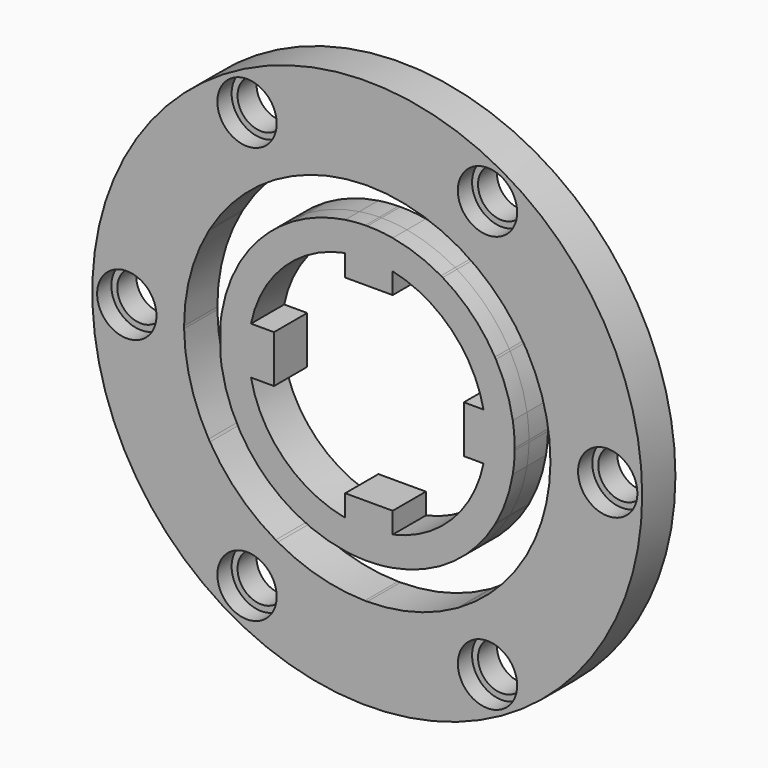
from build123d import *

# Parameters (mm, degrees)
F1_DEPTH      = 1.5
F1_DEPTH_BACK = 2
F0_R          = 23.1715188415
F14_D         = 4
F14_DEPTH     = 2.001
F15_D         = 5
F15_DEPTH     = 2
F15_TIP       = 1.5021515476


# Not quite as in the source:
# - the program builds the solid bodies; features that only make, move or delete a surface that nothing else refers to are left out


with BuildPart() as f1:
    # F0 (on Front) → F1 (new body, two sides)
    with BuildSketch(Plane.XZ) as f1_sk:
        with BuildLine():
            ThreePointArc((-9.7979589711, 2), (-7.0199538443, 7.1218149389), (-1.8586532747, 9.8257522869))
            Line((-1.8586532747, 9.8257522869), (-1.8586532747, 12.2861632234))
            ThreePointArc((-1.8586532747, 12.2861632234), (-4.1072121765, 11.7275405301), (-6.2129783266, 10.761194128))
            ThreePointArc((-6.2129783266, 10.761194128), (-6.2850915316, 10.7161183391), (-6.3596317791, 10.6751806721))
            ThreePointArc((-6.3596317791, 10.6751806721), (-8.7864782122, 8.7864782122), (-10.6751806721, 6.3596317791))
            ThreePointArc((-10.6751806721, 6.3596317791), (-10.7161183391, 6.2850915316), (-10.761194128, 6.2129783266))
            ThreePointArc((-10.761194128, 6.2129783266), (-11.7036993668, 4.174664044), (-12.2639471113, 2))
            Line((-12.2639471113, 2), (-9.7979589711, 2))
        make_face()
        with BuildLine():
            ThreePointArc((-9.7979589711, -2), (-10, 0), (-9.7979589711, 2))
            Line((-9.7979589711, 2), (-12.2639471113, 2))
            ThreePointArc((-12.2639471113, 2), (-12.3163951558, 1.6464534963), (-12.3586532747, 1.2915448051))
            Line((-12.3586532747, 1.2915448051), (-12.3586532747, -1.2915448051))
            ThreePointArc((-12.3586532747, -1.2915448051), (-12.3163951558, -1.6464534963), (-12.2639471113, -2))
            Line((-12.2639471113, -2), (-9.7979589711, -2))
        make_face()
        with BuildLine():
            Line((-7.8586532747, 2), (-9.7979589711, 2))
            ThreePointArc((-9.7979589711, 2), (-10, 0), (-9.7979589711, -2))
            Line((-9.7979589711, -2), (-7.8586532747, -2))
            Line((-7.8586532747, -2), (-7.8586532747, 2))
        make_face()
        with BuildLine():
            Line((-1.8586532747, -12.2861632234), (-1.8586532747, -9.8257522869))
            ThreePointArc((-1.8586532747, -9.8257522869), (-7.0199538443, -7.1218149389), (-9.7979589711, -2))
            Line((-9.7979589711, -2), (-12.2639471113, -2))
            ThreePointArc((-12.2639471113, -2), (-11.7036993668, -4.174664044), (-10.761194128, -6.2129783266))
            ThreePointArc((-10.761194128, -6.2129783266), (-10.7161183391, -6.2850915316), (-10.6751806721, -6.3596317791))
            ThreePointArc((-10.6751806721, -6.3596317791), (-8.7261627517, -8.8463824459), (-6.2129783266, -10.761194128))
            ThreePointArc((-6.2129783266, -10.761194128), (-6.1378849458, -10.801108101), (-6.0651617625, -10.8451930155))
            ThreePointArc((-6.0651617625, -10.8451930155), (-4.02688589, -11.7553642554), (-1.8586532747, -12.2861632234))
        make_face()
        with BuildLine():
            Line((2.1413467253, -12.2400585354), (2.1413467253, -9.7680414722))
            ThreePointArc((2.1413467253, -9.7680414722), (0.144262023, -9.9989593693), (-1.8586532747, -9.8257522869))
            Line((-1.8586532747, -9.8257522869), (-1.8586532747, -12.2861632234))
            ThreePointArc((-1.8586532747, -12.2861632234), (-1.0166984011, -12.3842934037), (-0.1700123434, -12.4247935416))
            ThreePointArc((-0.1700123434, -12.4247935416), (-0.0849897619, -12.4229764774), (0, -12.4259566532))
            ThreePointArc((0, -12.4259566532), (1.0747004127, -12.3793948871), (2.1413467253, -12.2400585354))
        make_face()
        with BuildLine():
            ThreePointArc((-1.8586532747, -9.8257522869), (0.144262023, -9.9989593693), (2.1413467253, -9.7680414722))
            Line((2.1413467253, -9.7680414722), (2.1413467253, -8))
            Line((2.1413467253, -8), (-1.8586532747, -8))
            Line((-1.8586532747, -8), (-1.8586532747, -9.8257522869))
        make_face()
        with BuildLine():
            Line((12.2639471113, -2), (9.7979589711, -2))
            ThreePointArc((9.7979589711, -2), (7.1219640694, -7.0198025466), (2.1413467253, -9.7680414722))
            Line((2.1413467253, -9.7680414722), (2.1413467253, -12.2400585354))
            ThreePointArc((2.1413467253, -12.2400585354), (4.1621037763, -11.708171971), (6.0651617625, -10.8451930155))
            ThreePointArc((6.0651617625, -10.8451930155), (6.1378849458, -10.801108101), (6.2129783266, -10.761194128))
            ThreePointArc((6.2129783266, -10.761194128), (8.7864782122, -8.7864782122), (10.761194128, -6.2129783266))
            ThreePointArc((10.761194128, -6.2129783266), (10.801108101, -6.1378849458), (10.8451930155, -6.0651617625))
            ThreePointArc((10.8451930155, -6.0651617625), (11.7319851001, -4.0944992807), (12.2639471113, -2))
        make_face()
        with BuildLine():
            ThreePointArc((9.7979589711, 2), (9.9493615301, 1.0050896201), (10, 0))
            ThreePointArc((10, 0), (9.9493615301, -1.0050896201), (9.7979589711, -2))
            Line((9.7979589711, -2), (12.2639471113, -2))
            ThreePointArc((12.2639471113, -2), (12.3782346262, -1.0879826681), (12.4247935416, -0.1700123434))
            ThreePointArc((12.4247935416, -0.1700123434), (12.4229764774, -0.0849897619), (12.4259566532, 0))
            ThreePointArc((12.4259566532, 0), (12.385388043, 1.0032755219), (12.2639471113, 2))
            Line((12.2639471113, 2), (9.7979589711, 2))
        make_face()
        with BuildLine():
            ThreePointArc((9.7979589711, -2), (9.9493615301, -1.0050896201), (10, 0))
            ThreePointArc((10, 0), (9.9493615301, 1.0050896201), (9.7979589711, 2))
            Line((9.7979589711, 2), (8.1413467253, 2))
            Line((8.1413467253, 2), (8.1413467253, -2))
            Line((8.1413467253, -2), (9.7979589711, -2))
        make_face()
        with BuildLine():
            ThreePointArc((2.1413467253, 9.7680414722), (7.1219640694, 7.0198025466), (9.7979589711, 2))
            Line((9.7979589711, 2), (12.2639471113, 2))
            ThreePointArc((12.2639471113, 2), (11.7319851001, 4.0944992807), (10.8451930155, 6.0651617625))
            ThreePointArc((10.8451930155, 6.0651617625), (10.801108101, 6.1378849458), (10.761194128, 6.2129783266))
            ThreePointArc((10.761194128, 6.2129783266), (8.8463824459, 8.7261627517), (6.3596317791, 10.6751806721))
            ThreePointArc((6.3596317791, 10.6751806721), (6.2850915316, 10.7161183391), (6.2129783266, 10.761194128))
            ThreePointArc((6.2129783266, 10.761194128), (4.2421040478, 11.6794243007), (2.1413467253, 12.2400585354))
            Line((2.1413467253, 12.2400585354), (2.1413467253, 9.7680414722))
        make_face()
        with BuildLine():
            ThreePointArc((-1.8586532747, 9.8257522869), (0.144262023, 9.9989593693), (2.1413467253, 9.7680414722))
            Line((2.1413467253, 9.7680414722), (2.1413467253, 12.2400585354))
            ThreePointArc((2.1413467253, 12.2400585354), (1.0747004127, 12.3793948871), (0, 12.4259566532))
            ThreePointArc((0, 12.4259566532), (-0.0849897619, 12.4229764774), (-0.1700123434, 12.4247935416))
            ThreePointArc((-0.1700123434, 12.4247935416), (-1.0166984011, 12.3842934037), (-1.8586532747, 12.2861632234))
            Line((-1.8586532747, 12.2861632234), (-1.8586532747, 9.8257522869))
        make_face()
        with BuildLine():
            Line((2.1413467253, 8), (2.1413467253, 9.7680414722))
            ThreePointArc((2.1413467253, 9.7680414722), (0.144262023, 9.9989593693), (-1.8586532747, 9.8257522869))
            Line((-1.8586532747, 9.8257522869), (-1.8586532747, 8))
            Line((-1.8586532747, 8), (2.1413467253, 8))
        make_face()
    extrude(amount=F1_DEPTH)
    extrude(f1_sk.sketch, amount=-F1_DEPTH_BACK)


with BuildPart() as f1b:
    # F0 (on Front) → F1, piece 2 (new body, two sides)
    with BuildSketch(Plane.XZ) as f1_2_sk:
        Circle(F0_R)
        Polygon((10.1330032136, 17.5508763992), (20.2660064272, 0), (10.1330032136, -17.5508763992), (-10.1330032136, -17.5508763992), (-20.2660064272, 0), (-10.1330032136, 17.5508763992), align=None, mode=Mode.SUBTRACT)
        Polygon((10.1330032136, -17.5508763992), (20.2660064272, 0), (10.1330032136, 17.5508763992), (-10.1330032136, 17.5508763992), (-20.2660064272, 0), (-10.1330032136, -17.5508763992), align=None)
        with BuildLine():
            ThreePointArc((13.3670856415, 7.7174904934), (13.4224746928, 7.6275141941), (13.4714253931, 7.5338792094))
            ThreePointArc((13.4714253931, 7.5338792094), (14.936027465, 3.8927781375), (15.4349809868, 0))
            ThreePointArc((15.4349809868, 0), (15.4379611627, -0.1056162866), (15.4335362203, -0.2111819122))
            ThreePointArc((15.4335362203, -0.2111819122), (14.9090467635, -3.9948670402), (13.4714253931, -7.5338792094))
            ThreePointArc((13.4714253931, -7.5338792094), (13.4224746928, -7.6275141941), (13.3670856415, -7.7174904934))
            ThreePointArc((13.3670856415, -7.7174904934), (10.9141797233, -10.9141797233), (7.7174904934, -13.3670856415))
            ThreePointArc((7.7174904934, -13.3670856415), (7.6275141941, -13.4224746928), (7.5338792094, -13.4714253931))
            ThreePointArc((7.5338792094, -13.4714253931), (3.8927781375, -14.936027465), (0, -15.4349809868))
            ThreePointArc((0, -15.4349809868), (-0.1056162866, -15.4379611627), (-0.2111819122, -15.4335362203))
            ThreePointArc((-0.2111819122, -15.4335362203), (-3.9948670402, -14.9090467635), (-7.5338792094, -13.4714253931))
            ThreePointArc((-7.5338792094, -13.4714253931), (-7.6275141941, -13.4224746928), (-7.7174904934, -13.3670856415))
            ThreePointArc((-7.7174904934, -13.3670856415), (-10.8392584909, -10.9885901476), (-13.2602434809, -7.899657011))
            ThreePointArc((-13.2602434809, -7.899657011), (-13.3168584062, -7.8104469685), (-13.3670856415, -7.7174904934))
            ThreePointArc((-13.3670856415, -7.7174904934), (-14.8813682851, -4.0967689742), (-15.4335362203, -0.2111819122))
            ThreePointArc((-15.4335362203, -0.2111819122), (-15.4379611627, -0.1056162866), (-15.4349809868, 0))
            ThreePointArc((-15.4349809868, 0), (-14.9090467635, 3.9948670402), (-13.3670856415, 7.7174904934))
            ThreePointArc((-13.3670856415, 7.7174904934), (-13.3168584062, 7.8104469685), (-13.2602434809, 7.899657011))
            ThreePointArc((-13.2602434809, 7.899657011), (-10.9141797233, 10.9141797233), (-7.899657011, 13.2602434809))
            ThreePointArc((-7.899657011, 13.2602434809), (-7.8104469685, 13.3168584062), (-7.7174904934, 13.3670856415))
            ThreePointArc((-7.7174904934, 13.3670856415), (-4.0967689742, 14.8813682851), (-0.2111819122, 15.4335362203))
            ThreePointArc((-0.2111819122, 15.4335362203), (-0.1056162866, 15.4379611627), (0, 15.4349809868))
            ThreePointArc((0, 15.4349809868), (3.9948670402, 14.9090467635), (7.7174904934, 13.3670856415))
            ThreePointArc((7.7174904934, 13.3670856415), (7.8104469685, 13.3168584062), (7.899657011, 13.2602434809))
            ThreePointArc((7.899657011, 13.2602434809), (10.9885901476, 10.8392584909), (13.3670856415, 7.7174904934))
        make_face(mode=Mode.SUBTRACT)
    extrude(amount=F1_DEPTH)
    extrude(f1_2_sk.sketch, amount=-F1_DEPTH_BACK)

    # F14 (through all, one way)
    with BuildSketch(Plane.XZ):
        with Locations((-20.2660064272, 0), (-10.1330032136, -17.5508763992), (10.1330032136, -17.5508763992), (20.2660064272, 0), (10.1330032136, 17.5508763992), (-10.1330032136, 17.5508763992)):
            Circle(F14_D / 2)
    extrude(amount=-F14_DEPTH, mode=Mode.SUBTRACT)

    # F15 (one way)
    with BuildSketch(Plane(origin=(0, 0, 0), x_dir=(1, 0, 0), z_dir=(0, 1, 0))):
        with Locations((10.1330032136, 17.5508763992), (-10.1330032136, 17.5508763992), (-20.2660064272, 0), (-10.1330032136, -17.5508763992), (10.1330032136, -17.5508763992), (20.2660064272, 0)):
            Circle(F15_D / 2)
    extrude(amount=-F15_DEPTH, mode=Mode.SUBTRACT)
    with Locations(Plane(origin=(0, 0, 0), x_dir=(1, 0, 0), z_dir=(0, 1, 0))):
        with Locations((10.1330032136, 17.5508763992), (-10.1330032136, 17.5508763992), (-20.2660064272, 0), (-10.1330032136, -17.5508763992), (10.1330032136, -17.5508763992), (20.2660064272, 0)):
            with Locations((0, 0, -(F15_DEPTH + F15_TIP / 2))):  # 118° drill point
                Cone(0, F15_D / 2, F15_TIP, mode=Mode.SUBTRACT)


solid = Compound([f1.part, f1b.part])
